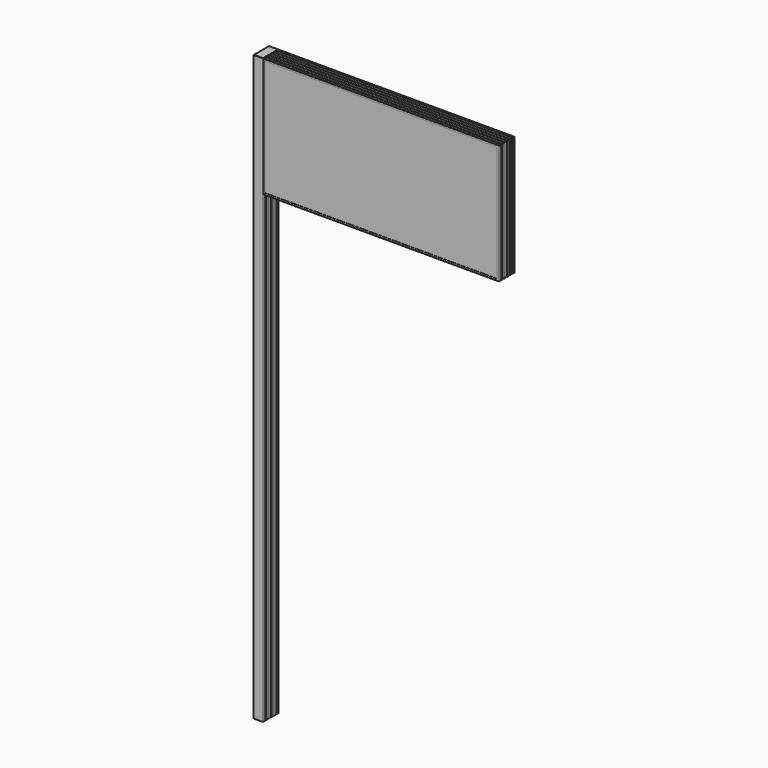
from build123d import *

# Parameters (mm, degrees)
F0_W          = 50
F0_H          = 3020
F1_DEPTH      = 100
F2_W          = 1220
F2_H          = 100
F3_DEPTH      = 620
F2_W_2        = 5000
F4_W          = 1200
F4_H          = 600
F4_W_2        = 4980
F5_DEPTH      = 100.001
F6_W          = 8
F6_H          = 2
F7_DEPTH      = 7540.001
F8_W          = 2
F8_H          = 8
F9_DEPTH      = 3020.001
F11_W         = 4980
F11_H         = 600
F12_DEPTH     = 98
F11_W_2       = 1200
F13_R         = 1.9999
F13_2_R       = 1.9999
F13_3_R       = 1.9999
F13_4_R       = 1.9999
F14_W         = 2
F14_H         = 8
F15_DEPTH     = 3020.001
F16_T1_DEPTH  = 3025
F16_T4_ANGLE  = 90
F16_T6_ANGLE  = 90
F16_T8_ANGLE  = 90
F16_T10_ANGLE = 90


# Not quite as in the source:
# - a fillet or chamfer that OpenCascade refuses, or shapes differently, is made with other operations: its cross-section is extruded or revolved along the edge and cut away or added
# - a fillet or chamfer is up to 0.001 mm smaller than in the source, because OpenCascade refuses the exact size


with BuildPart() as f1:
    # F0 (on Front) → F1 (new body)
    with BuildSketch(Plane.XZ):
        with Locations((-2525, -1510)):
            Rectangle(F0_W, F0_H)
    extrude(amount=F1_DEPTH)


with BuildPart() as f1b:
    # F0 (on Front) → F1, piece 2 (new body)
    with BuildSketch(Plane.XZ):
        with Locations((2525, -1510)):
            Rectangle(F0_W, F0_H)
    extrude(amount=F1_DEPTH)

    # F13 (radius 2 in the source; OpenCascade refuses exactly that, so slightly less here)
    f13_edges = [f1b.edges().sort_by_distance(p)[0] for p in [
        (2550, -50, 0),
        (2500, -50, 0),
        (2525, 0, 0),
        (2525, -100, 0),
    ]]
    fillet(f13_edges, radius=F13_R)


with BuildPart() as f3:
    # F2 (on face) → F3 (new body)
    with BuildSketch(Plane.XY):
        with Locations((-3160, -50)):
            Rectangle(F2_W, F2_H)
    extrude(amount=-F3_DEPTH)


with BuildPart() as f3b:
    # F2 (on face) → F3, piece 2 (new body)
    with BuildSketch(Plane.XY):
        with Locations((0, -50)):
            Rectangle(F2_W_2, F2_H)
    extrude(amount=-F3_DEPTH)


with BuildPart() as f3c:
    # F2 (on face) → F3, piece 3 (new body)
    with BuildSketch(Plane.XY):
        with Locations((3160, -50)):
            Rectangle(F2_W, F2_H)
    extrude(amount=-F3_DEPTH)


with BuildPart() as f5_tool:
    # F4 (on face) → F5 (new body, through all)
    with BuildSketch(Plane.XZ.offset(100)):
        with Locations((-3160, -310)):
            Rectangle(F4_W, F4_H)
        with Locations((0, -310)):
            Rectangle(F4_W_2, F4_H)
        with Locations((3160, -310)):
            Rectangle(F4_W, F4_H)
    extrude(amount=-F5_DEPTH)


with BuildPart() as f3_1:
    add(f3.part)

    # F5: cut by f5_tool
    add(f5_tool.part, mode=Mode.SUBTRACT)


with BuildPart() as f3b_1:
    add(f3b.part)

    # F5: cut by f5_tool
    add(f5_tool.part, mode=Mode.SUBTRACT)


with BuildPart() as f3c_1:
    add(f3c.part)

    # F5: cut by f5_tool
    add(f5_tool.part, mode=Mode.SUBTRACT)


with BuildPart() as f7_tool:
    # F6 (on face) → F7 (new body, through all)
    with BuildSketch(Plane(origin=(-3770, 0, 0), x_dir=(0, -1, 0), z_dir=(-1, 0, 0))):
        with Locations((14, -1)):
            Rectangle(F6_W, F6_H)
        with Locations((32, -1)):
            Rectangle(F6_W, F6_H)
        with Locations((50, -1)):
            Rectangle(F6_W, F6_H)
        with Locations((68, -1)):
            Rectangle(F6_W, F6_H)
        with Locations((86, -1)):
            Rectangle(F6_W, F6_H)
        with Locations((86, -619)):
            Rectangle(F6_W, F6_H)
        with Locations((68, -619)):
            Rectangle(F6_W, F6_H)
        with Locations((14, -619)):
            Rectangle(F6_W, F6_H)
        with Locations((32, -619)):
            Rectangle(F6_W, F6_H)
        with Locations((50, -619)):
            Rectangle(F6_W, F6_H)
    extrude(amount=-F7_DEPTH)


with BuildPart() as f1_1:
    add(f1.part)

    # F7: cut by f7_tool
    add(f7_tool.part, mode=Mode.SUBTRACT)


with BuildPart() as f3_2:
    add(f3_1.part)

    # F7: cut by f7_tool
    add(f7_tool.part, mode=Mode.SUBTRACT)


with BuildPart() as f3b_2:
    add(f3b_1.part)

    # F7: cut by f7_tool
    add(f7_tool.part, mode=Mode.SUBTRACT)

    # F13#3 (radius 2 in the source; OpenCascade refuses exactly that, so slightly less here)
    f13_3_edges = [f3b_2.edges().sort_by_distance(p)[0] for p in [
        (2500, -41, 0),
        (2500, -23, 0),
        (2500, -5, 0),
        (2500, -59, 0),
        (2500, -77, 0),
        (2500, -95, 0),
        (2500, -86, -2),
        (2500, -68, -2),
        (2500, -50, -2),
        (2500, -32, -2),
        (2500, -14, -2),
        (2500, -86, -618),
        (2500, -68, -618),
        (2500, -50, -618),
        (2500, -32, -618),
        (2500, -14, -618),
        (-2500, -5, -620),
        (-2500, -23, -620),
        (-2500, -32, -618),
        (-2500, -41, -620),
        (-2500, -50, -618),
        (-2500, -59, -620),
        (-2500, -68, -618),
        (-2500, -77, -620),
        (-2500, -86, -618),
        (-2500, -95, -620),
        (-2500, -14, -618),
        (-2500, -95, 0),
        (-2500, -77, 0),
        (-2500, -59, 0),
        (-2500, -68, -2),
        (-2500, -86, -2),
        (-2500, -50, -2),
        (-2500, -41, 0),
        (-2500, -32, -2),
        (-2500, -23, 0),
        (-2500, -14, -2),
        (-2500, -5, 0),
    ]]
    fillet(f13_3_edges, radius=F13_3_R)


with BuildPart() as f3c_2:
    add(f3c_1.part)

    # F7: cut by f7_tool
    add(f7_tool.part, mode=Mode.SUBTRACT)


with BuildPart() as f9_tool:
    # F8 (on face) → F9 (new body, through all)
    with BuildSketch(Plane.XY):
        with Locations((-3769, -86)):
            Rectangle(F8_W, F8_H)
        with Locations((-3769, -68)):
            Rectangle(F8_W, F8_H)
        with Locations((-3769, -50)):
            Rectangle(F8_W, F8_H)
        with Locations((-3769, -32)):
            Rectangle(F8_W, F8_H)
        with Locations((-3769, -14)):
            Rectangle(F8_W, F8_H)
        with Locations((3769, -68)):
            Rectangle(F8_W, F8_H)
        with Locations((3769, -32)):
            Rectangle(F8_W, F8_H)
        with Locations((3769, -86)):
            Rectangle(F8_W, F8_H)
        with Locations((3769, -50)):
            Rectangle(F8_W, F8_H)
        with Locations((3769, -14)):
            Rectangle(F8_W, F8_H)
    extrude(amount=-F9_DEPTH)


with BuildPart() as f3_3:
    add(f3_2.part)

    # F9: cut by f9_tool
    add(f9_tool.part, mode=Mode.SUBTRACT)

    # F13#2 (radius 2 in the source; OpenCascade refuses exactly that, so slightly less here)
    f13_2_edges = [f3_3.edges().sort_by_distance(p)[0] for p in [
        (-2550, -5, -620),
        (-2550, -14, -618),
        (-2550, -23, -620),
        (-2550, -32, -618),
        (-2550, -41, -620),
        (-2550, -50, -618),
        (-2550, -59, -620),
        (-2550, -68, -618),
        (-2550, -77, -620),
        (-2550, -86, -618),
        (-2550, -95, -620),
        (-3770, -95, -620),
        (-3768, -86, -618),
        (-3770, -77, -620),
        (-3768, -68, -618),
        (-3770, -59, -620),
        (-3768, -50, -618),
        (-3770, -41, -620),
        (-3768, -32, -618),
        (-3770, -23, -620),
        (-3768, -14, -618),
        (-3770, -5, -620),
        (-3770, -95, 0),
        (-3768, -86, -2),
        (-3770, -77, 0),
        (-3768, -68, -2),
        (-3770, -59, 0),
        (-3768, -50, -2),
        (-3770, -41, 0),
        (-3768, -32, -2),
        (-3770, -23, 0),
        (-3768, -14, -2),
        (-3770, -5, 0),
        (-2550, -95, 0),
        (-2550, -77, 0),
        (-2550, -59, 0),
        (-2550, -41, 0),
        (-2550, -23, 0),
        (-2550, -5, 0),
        (-2550, -14, -2),
        (-2550, -32, -2),
        (-2550, -50, -2),
        (-2550, -68, -2),
        (-2550, -86, -2),
    ]]
    fillet(f13_2_edges, radius=F13_2_R)


with BuildPart() as f3c_3:
    add(f3c_2.part)

    # F9: cut by f9_tool
    add(f9_tool.part, mode=Mode.SUBTRACT)

    # F13#4 (radius 2 in the source; OpenCascade refuses exactly that, so slightly less here)
    f13_4_edges = [f3c_3.edges().sort_by_distance(p)[0] for p in [
        (3770, -5, 0),
        (3770, -23, 0),
        (3770, -41, 0),
        (3770, -59, 0),
        (3770, -77, 0),
        (3770, -95, 0),
        (3768, -86, -2),
        (3768, -68, -2),
        (3768, -50, -2),
        (3768, -32, -2),
        (3768, -14, -2),
        (2550, -5, 0),
        (2550, -23, 0),
        (2550, -41, 0),
        (2550, -59, 0),
        (2550, -95, 0),
        (2550, -77, 0),
        (2550, -86, -2),
        (2550, -68, -2),
        (2550, -50, -2),
        (2550, -32, -2),
        (2550, -14, -2),
        (3770, -5, -620),
        (3768, -14, -618),
        (3770, -23, -620),
        (3768, -32, -618),
        (3770, -41, -620),
        (3768, -50, -618),
        (3770, -59, -620),
        (3768, -68, -618),
        (3770, -77, -620),
        (3768, -86, -618),
        (3770, -95, -620),
        (2550, -5, -620),
        (2550, -14, -618),
        (2550, -23, -620),
        (2550, -32, -618),
        (2550, -41, -620),
        (2550, -50, -618),
        (2550, -59, -620),
        (2550, -68, -618),
        (2550, -77, -620),
        (2550, -86, -618),
        (2550, -95, -620),
        (2550, -100, -310),
        (2550, 0, -310),
        (3770, 0, -310),
        (3160, 0, 0),
        (3160, 0, -620),
        (3160, -100, -620),
        (3770, -100, -310),
        (3160, -100, 0),
    ]]
    fillet(f13_4_edges, radius=F13_4_R)


with BuildPart() as f12:
    # F11 (on offset) → F12 (new body, through all)
    with BuildSketch(Plane(origin=(0, -1, 0), x_dir=(-1, 0, 0), z_dir=(0, 1, 0))):
        with Locations((0, -310)):
            Rectangle(F11_W, F11_H)
    extrude(amount=-F12_DEPTH)


with BuildPart() as f12b:
    # F11 (on offset) → F12, piece 2 (new body, through all)
    with BuildSketch(Plane(origin=(0, -1, 0), x_dir=(-1, 0, 0), z_dir=(0, 1, 0))):
        with Locations((-3160, -310)):
            Rectangle(F11_W_2, F11_H)
    extrude(amount=-F12_DEPTH)


with BuildPart() as f12c:
    # F11 (on offset) → F12, piece 3 (new body, through all)
    with BuildSketch(Plane(origin=(0, -1, 0), x_dir=(-1, 0, 0), z_dir=(0, 1, 0))):
        with Locations((3160, -310)):
            Rectangle(F11_W_2, F11_H)
    extrude(amount=-F12_DEPTH)


with BuildPart() as f15_tool:
    # F14 (on face) → F15 (new body, through all)
    with BuildSketch(Plane(origin=(0, 0, -3020), x_dir=(1, 0, 0), z_dir=(0, 0, -1))):
        with Locations((-2549, 86)):
            Rectangle(F14_W, F14_H)
        with Locations((-2549, 14)):
            Rectangle(F14_W, F14_H)
        with Locations((-2549, 32)):
            Rectangle(F14_W, F14_H)
        with Locations((-2549, 50)):
            Rectangle(F14_W, F14_H)
        with Locations((-2549, 68)):
            Rectangle(F14_W, F14_H)
        with Locations((-2501, 32)):
            Rectangle(F14_W, F14_H)
        with Locations((-2501, 50)):
            Rectangle(F14_W, F14_H)
        with Locations((-2501, 14)):
            Rectangle(F14_W, F14_H)
        with Locations((-2501, 86)):
            Rectangle(F14_W, F14_H)
        with Locations((-2501, 68)):
            Rectangle(F14_W, F14_H)
        with Locations((2501, 50)):
            Rectangle(F14_W, F14_H)
        with Locations((2501, 86)):
            Rectangle(F14_W, F14_H)
        with Locations((2501, 32)):
            Rectangle(F14_W, F14_H)
        with Locations((2501, 68)):
            Rectangle(F14_W, F14_H)
        with Locations((2501, 14)):
            Rectangle(F14_W, F14_H)
        with Locations((2549, 68)):
            Rectangle(F14_W, F14_H)
        with Locations((2549, 14)):
            Rectangle(F14_W, F14_H)
        with Locations((2549, 50)):
            Rectangle(F14_W, F14_H)
        with Locations((2549, 32)):
            Rectangle(F14_W, F14_H)
        with Locations((2549, 86)):
            Rectangle(F14_W, F14_H)
    extrude(amount=-F15_DEPTH)


with BuildPart() as f1_2:
    add(f1_1.part)

    # F15: cut by f15_tool
    add(f15_tool.part, mode=Mode.SUBTRACT)


with BuildPart() as f1b_1:
    add(f1b.part)

    # F15: cut by f15_tool
    add(f15_tool.part, mode=Mode.SUBTRACT)

    # F16: fillet of radius 2 on 6 edges, made by hand

    # F16_s2 → F16_t1 (cut)
    with BuildSketch(Plane.XY.offset(-3025)):
        with BuildLine():
            ThreePointArc((2502, 0), (2500.5857864376, -0.5857864376), (2500, -2))
            Line((2500, -2), (2500, 0))
            Line((2500, 0), (2502, 0))
        make_face()
        with BuildLine():
            ThreePointArc((2502, -100), (2500.5857864376, -99.4142135624), (2500, -98))
            Line((2500, -98), (2500, -100))
            Line((2500, -100), (2502, -100))
        make_face()
        with BuildLine():
            ThreePointArc((2550, -2), (2549.4142135624, -0.5857864376), (2548, 0))
            Line((2548, 0), (2550, 0))
            Line((2550, 0), (2550, -2))
        make_face()
        with BuildLine():
            ThreePointArc((2550, -98), (2549.4142135624, -99.4142135624), (2548, -100))
            Line((2548, -100), (2550, -100))
            Line((2550, -100), (2550, -98))
        make_face()
    extrude(amount=F16_T1_DEPTH, mode=Mode.SUBTRACT)

    # F16_s3 → F16_t4 (revolve, cut)
    with BuildSketch(Plane.XZ.offset(2)):
        with BuildLine():
            ThreePointArc((2548.0001, 0), (2549.4142428517, -0.5857571483), (2550, -1.9999))
            Line((2550, -1.9999), (2550, 0))
            Line((2550, 0), (2548.0001, 0))
        make_face()
    revolve(axis=Axis((2548, -2, 0), (0, 0, 1)), revolution_arc=F16_T4_ANGLE, mode=Mode.SUBTRACT)

    # F16_s5 → F16_t6 (revolve, cut)
    with BuildSketch(Plane.YZ.offset(2548)):
        with BuildLine():
            ThreePointArc((-98.0001, 0), (-99.4142428517, -0.5857571483), (-100, -1.9999))
            Line((-100, -1.9999), (-100, 0))
            Line((-100, 0), (-98.0001, 0))
        make_face()
    revolve(axis=Axis((2548, -98, 0), (0, 0, 1)), revolution_arc=F16_T6_ANGLE, mode=Mode.SUBTRACT)

    # F16_s7 → F16_t8 (revolve, cut)
    with BuildSketch(Plane.XZ.offset(98)):
        with BuildLine():
            ThreePointArc((2501.9999, 0), (2500.5857571483, -0.5857571483), (2500, -1.9999))
            Line((2500, -1.9999), (2500, 0))
            Line((2500, 0), (2501.9999, 0))
        make_face()
    revolve(axis=Axis((2502, -98, 0), (0, 0, 1)), revolution_arc=F16_T8_ANGLE, mode=Mode.SUBTRACT)

    # F16_s9 → F16_t10 (revolve, cut)
    with BuildSketch(Plane.YZ.offset(2502)):
        with BuildLine():
            ThreePointArc((-1.9999, 0), (-0.5857571483, -0.5857571483), (0, -1.9999))
            Line((0, -1.9999), (0, 0))
            Line((0, 0), (-1.9999, 0))
        make_face()
    revolve(axis=Axis((2502, -2, 0), (0, 0, 1)), revolution_arc=F16_T10_ANGLE, mode=Mode.SUBTRACT)


solid = Compound([f3c_3.part, f12b.part, f1b_1.part])
